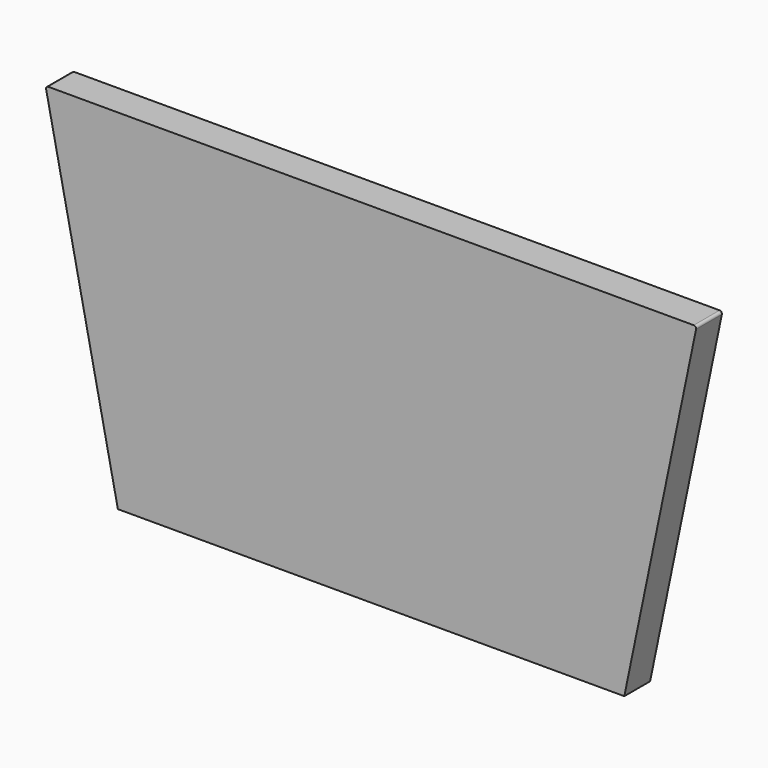
from build123d import *

# Parameters (mm, degrees)
F1_DEPTH = 86.36


# Not quite as in the source:
# - a feature of the source that left no trace in its solid (it failed there, or was rolled back) is left out


with BuildPart() as f1:
    # F0 (on Front) → F1 (new body)
    with BuildSketch(Plane.XZ):
        with BuildLine():
            Line((699.6463771647, 476.5957295895), (-1027.3060432158, 476.5957295895))
            ThreePointArc((-1027.3060432158, 476.5957295895), (-1032.2305974455, 474.2546278967), (-1033.5240076617, 468.9575455385))
            Line((-1033.5240076617, 468.9575455385), (-841.4893746376, -457.9787254334))
            Line((-841.4893746376, -457.9787254333), (513.829767704, -457.9787254333))
            Line((513.829767704, -457.9787254333), (705.8643416894, 468.9575459187))
            ThreePointArc((705.8643416894, 468.9575459187), (704.5709312719, 474.2546280473), (699.6463771647, 476.5957295895))
        make_face()
    extrude(amount=F1_DEPTH)


solid = f1.part
